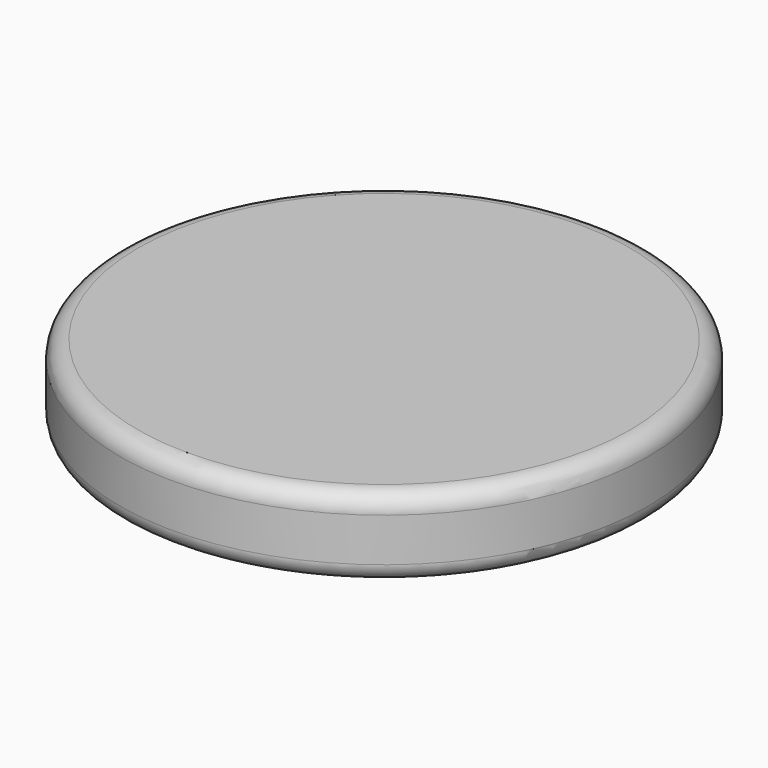
from build123d import *

# Parameters (mm, degrees)
F0_R     = 75.3277173883
F1_DEPTH = 22.606
F2_R     = 5.08
F3_R     = 5.08


with BuildPart() as f1:
    # F0 (on Top) → F1 (new body)
    with BuildSketch(Plane.XY):
        Circle(F0_R)
    extrude(amount=F1_DEPTH)

    # F2
    f2_edges = [f1.edges().sort_by_distance(p)[0] for p in [
        (-75.327717, 0, 0),
    ]]
    fillet(f2_edges, radius=F2_R)

    # F3
    f3_edges = [f1.edges().sort_by_distance(p)[0] for p in [
        (75.327717, 0, 13.843),
        (-75.327717, 0, 5.08),
        (-75.327717, 0, 22.606),
    ]]
    fillet(f3_edges, radius=F3_R)


solid = f1.part
